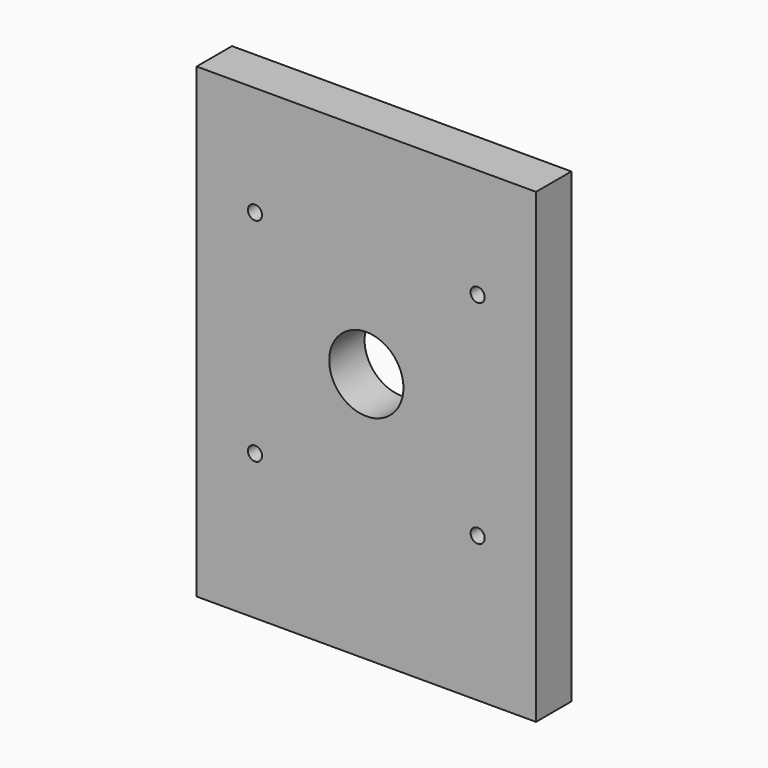
from build123d import *

# Parameters (mm, degrees)
F0_W     = 76.2
F0_H     = 104.775
F0_R     = 1.5875
F0_R_2   = 8.334375
F1_DEPTH = 9.921875


# Not quite as in the source:
# - a length typed as a fraction of an inch, garbled in the dataset ("3 / 203.2 mm" for 3/8 in), is restored


with BuildPart() as f1:
    # F0 (on Front) → F1 (new body)
    with BuildSketch(Plane.XZ):
        with Locations((0, -3.96875)):
            Rectangle(F0_W, F0_H)
        with Locations((-25.003125, -23.8125)):
            Circle(F0_R, mode=Mode.SUBTRACT)
        with Locations((25.003125, -23.8125)):
            Circle(F0_R, mode=Mode.SUBTRACT)
        with Locations((-25.003125, 23.8125)):
            Circle(F0_R, mode=Mode.SUBTRACT)
        Circle(F0_R_2, mode=Mode.SUBTRACT)
        with Locations((25.003125, 23.8125)):
            Circle(F0_R, mode=Mode.SUBTRACT)
    extrude(amount=F1_DEPTH)


solid = f1.part
